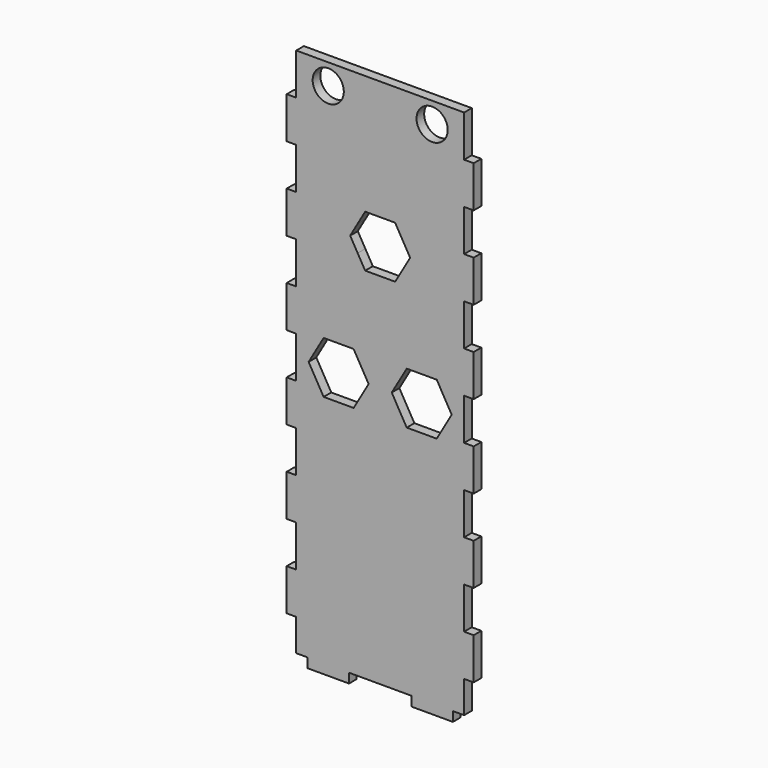
from build123d import *

# Parameters (mm, degrees)
F0_W     = 114.3
F0_H     = 330.2
F1_DEPTH = 5.842
F2_W     = 38.1
F2_H     = 5.842
F2_W_2   = 5.842
F2_H_2   = 25.4
F3_DEPTH = 25.4
F4_R     = 9.525
F5_DEPTH = 5.842


# Not quite as in the source:
# - a feature names something its author has since deleted; it is built from what else it names


with BuildPart() as f1:
    # F0 (on Front) → F1 (new body)
    with BuildSketch(Plane.XZ):
        with Locations((-25.4490938969, 91.3394362139)):
            Rectangle(F0_W, F0_H)
    extrude(amount=F1_DEPTH)

    # F2 (on face) → F3 (cut)
    with BuildSketch(Plane.XZ.offset(5.842)):
        Polygon((-82.5990938969, -73.7605637861), (-69.8990938969, -73.7605637861), (-69.8990938969, -67.9185637861), (-76.7570938969, -67.9185637861), (-76.7570938969, -48.3605637861), (-82.5990938969, -48.3605637861), align=None)
        with Locations((-25.4490938969, -70.8395637861)):
            Rectangle(F2_W, F2_H)
        Polygon((19.0009061031, -67.9185637861), (19.0009061031, -73.7605637861), (31.7009061031, -73.7605637861), (31.7009061031, -48.3605637861), (25.8589061031, -48.3605637861), (25.8589061031, -67.9185637861), align=None)
        with Locations((-79.6780938969, -10.2605637861)):
            Rectangle(F2_W_2, F2_H_2)
        with Locations((28.7799061031, -10.2605637861)):
            Rectangle(F2_W_2, F2_H_2)
        with Locations((-79.6780938969, 40.5394362139)):
            Rectangle(F2_W_2, F2_H_2)
        with Locations((28.7799061031, 40.5394362139)):
            Rectangle(F2_W_2, F2_H_2)
        with Locations((-79.6780938969, 91.3394362139)):
            Rectangle(F2_W_2, F2_H_2)
        with Locations((28.7799061031, 91.3394362139)):
            Rectangle(F2_W_2, F2_H_2)
        with Locations((-79.6780938969, 142.1394362139)):
            Rectangle(F2_W_2, F2_H_2)
        with Locations((28.7799061031, 142.1394362139)):
            Rectangle(F2_W_2, F2_H_2)
        with Locations((-79.6780938969, 192.9394362139)):
            Rectangle(F2_W_2, F2_H_2)
        with Locations((28.7799061031, 192.9394362139)):
            Rectangle(F2_W_2, F2_H_2)
        with Locations((28.7799061031, 243.7394362139)):
            Rectangle(F2_W_2, F2_H_2)
        with Locations((-79.6780938969, 243.7394362139)):
            Rectangle(F2_W_2, F2_H_2)
    extrude(amount=-F3_DEPTH, mode=Mode.SUBTRACT)

    # F4 (on face) → F5 (cut, through all)
    with BuildSketch(Plane.XZ.offset(5.842)):
        with BuildLine():
            ThreePointArc((-11.7009406501, 159.6019361475), (-10.1150214145, 163.4306838358), (-9.5740938969, 167.5394362139))
            ThreePointArc((-9.5740938969, 167.5394362139), (-10.1150214004, 171.6481885393), (-11.7009405957, 175.4769361859))
            ThreePointArc((-11.7009405957, 175.4769361859), (-17.5115938829, 181.2875894909), (-25.4490938969, 183.4144362139))
            ThreePointArc((-25.4490938969, 183.4144362139), (-33.3865937403, 181.2875895894), (-39.1972470011, 175.4769365272))
            ThreePointArc((-39.1972470011, 175.4769365272), (-41.3240938969, 167.5394362139), (-39.1972470011, 159.6019359006))
            ThreePointArc((-39.1972470011, 159.6019359006), (-33.3865937403, 153.7912828383), (-25.4490938969, 151.6644362139))
            ThreePointArc((-25.4490938969, 151.6644362139), (-17.5115939301, 153.7912829096), (-11.7009406501, 159.6019361475))
        make_face()
        with Locations((-57.1990938969, 243.7394362139)):
            Circle(F4_R)
        with Locations((6.3009061031, 243.7394362139)):
            Circle(F4_R)
        Polygon((-32.5182228501, 91.3394362139), (-41.6836583735, 107.2144362139), (-60.0145294203, 107.2144362139), (-69.1799649437, 91.3394362139), (-60.0145294203, 75.4644362139), (-41.6836583735, 75.4644362139), align=None)
        Polygon((18.2817771499, 91.3394362139), (9.1163416265, 107.2144362139), (-9.2145294203, 107.2144362139), (-18.3799649437, 91.3394362139), (-9.2145294203, 75.4644362139), (9.1163416265, 75.4644362139), align=None)
        with BuildLine():
            ThreePointArc((-39.1972470011, 175.4769365272), (-33.3865937403, 181.2875895894), (-25.4490938969, 183.4144362139))
            Line((-25.4490938969, 183.4144362139), (-34.6145294203, 183.4144362139))
            Line((-34.6145294203, 183.4144362139), (-39.1972470011, 175.4769365272))
        make_face()
        with BuildLine():
            ThreePointArc((-25.4490938969, 183.4144362139), (-17.5115938829, 181.2875894909), (-11.7009405957, 175.4769361859))
            Line((-11.7009405957, 175.4769361859), (-16.2836583735, 183.4144362139))
            Line((-16.2836583735, 183.4144362139), (-25.4490938969, 183.4144362139))
        make_face()
        with BuildLine():
            ThreePointArc((-11.7009405957, 175.4769361859), (-10.1150214004, 171.6481885393), (-9.5740938969, 167.5394362139))
            ThreePointArc((-9.5740938969, 167.5394362139), (-10.1150214145, 163.4306838358), (-11.7009406501, 159.6019361475))
            Line((-11.7009406501, 159.6019361475), (-7.1182228501, 167.5394362139))
            Line((-7.1182228501, 167.5394362139), (-11.7009405957, 175.4769361859))
        make_face()
        with BuildLine():
            Line((-16.2836583735, 151.6644362139), (-11.7009406501, 159.6019361475))
            ThreePointArc((-11.7009406501, 159.6019361475), (-17.5115939301, 153.7912829096), (-25.4490938969, 151.6644362139))
            Line((-25.4490938969, 151.6644362139), (-16.2836583735, 151.6644362139))
        make_face()
        with BuildLine():
            Line((-34.6145294203, 151.6644362139), (-25.4490938969, 151.6644362139))
            ThreePointArc((-25.4490938969, 151.6644362139), (-33.3865937403, 153.7912828383), (-39.1972470011, 159.6019359006))
            Line((-39.1972470011, 159.6019359006), (-34.6145294203, 151.6644362139))
        make_face()
        with BuildLine():
            ThreePointArc((-39.1972470011, 159.6019359006), (-41.3240938969, 167.5394362139), (-39.1972470011, 175.4769365272))
            Line((-39.1972470011, 175.4769365272), (-43.7799649437, 167.5394362139))
            Line((-43.7799649437, 167.5394362139), (-39.1972470011, 159.6019359006))
        make_face()
    extrude(amount=-F5_DEPTH, mode=Mode.SUBTRACT)


solid = f1.part
